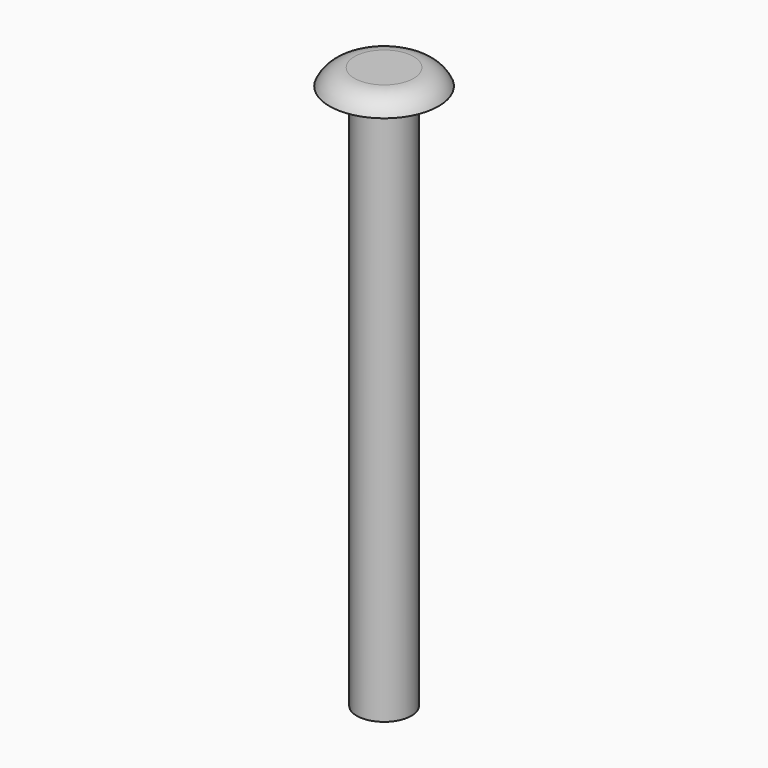
from build123d import *

# Parameters (mm, degrees)
F0_R     = 0.127
F1_DEPTH = 2.54
F2_R     = 0.254
F2_R_2   = 0.127
F3_DEPTH = 0.0762
F4_DEPTH = 0.0762


# Not quite as in the source:
# - a fillet or chamfer that OpenCascade refuses, or shapes differently, is made with other operations: its cross-section is extruded or revolved along the edge and cut away or added


with BuildPart() as f1:
    # F0 (on Top) → F1 (new body)
    with BuildSketch(Plane.XY):
        Circle(F0_R)
    extrude(amount=F1_DEPTH)

    # F2 (on face) → F3 (join)
    with BuildSketch(Plane.XY.offset(2.54)):
        Circle(F2_R)
        Circle(F2_R_2, mode=Mode.SUBTRACT)
    extrude(amount=F3_DEPTH)

    # F4 (add): a face of the model
    f4_faces = [f1.faces().sort_by_distance(p)[0] for p in [
        (0, 0, 2.54),
    ]]
    extrude(f4_faces, amount=F4_DEPTH)

    # F5: fillet of radius 0.127 on 1 edges, made by hand

    # F5_s1 → F5_t2 (revolve, cut)
    with BuildSketch(Plane.XZ):
        with BuildLine():
            ThreePointArc((0.254, 2.54), (0.2071633422, 2.5954558234), (0.1376025773, 2.6162))
            Line((0.1376025773, 2.6162), (0.254, 2.6162))
            Line((0.254, 2.6162), (0.254, 2.54))
        make_face()
    revolve(axis=Axis((0, 0, 2.6162), (0, 0, 1)), mode=Mode.SUBTRACT)


solid = f1.part
